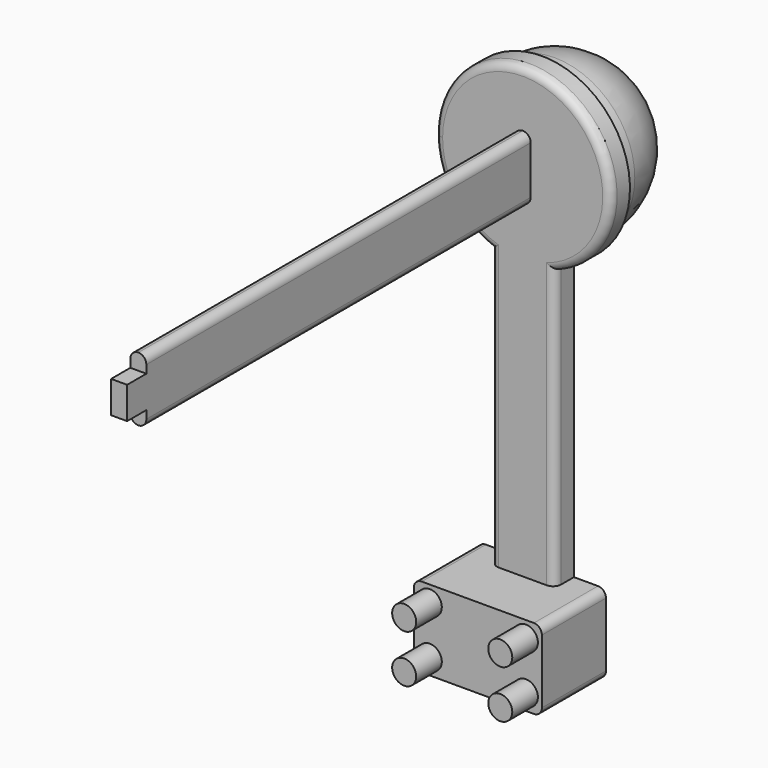
from build123d import *

# Parameters (mm, degrees)
F0_W      = 8
F0_H      = 5
F1_DEPTH  = 5
F2_R      = 0.75
F3_DEPTH  = 2
F4_W      = 4
F4_H      = 1.5
F5_DEPTH  = 23.5
F7_DEPTH  = 1.5
F8_W      = 1
F8_H      = 4
F9_DEPTH  = 30
F10_W     = 1
F10_H     = 2
F11_DEPTH = 1.5
F12_R     = 5
F13_DEPTH = 1
F15_ANGLE = 180
F16_R     = 0.49999
F17_R     = 0.5
F18_R     = 0.5


# Not quite as in the source:
# - a fillet or chamfer is up to 0.001 mm smaller than in the source, because OpenCascade refuses the exact size
# - a feature names something its author has since deleted; it is built from what else it names


with BuildPart() as f1:
    # F0 (on Front) → F1 (new body)
    with BuildSketch(Plane.XZ):
        Rectangle(F0_W, F0_H)
    extrude(amount=F1_DEPTH)

    # F2 (on face) → F3 (join)
    with BuildSketch(Plane.XZ.offset(5)):
        with Locations((-3, 1.5)):
            Circle(F2_R)
        with Locations((3, 1.5)):
            Circle(F2_R)
        with Locations((-3, -1.5)):
            Circle(F2_R)
        with Locations((3, -1.5)):
            Circle(F2_R)
    extrude(amount=F3_DEPTH)

    # F4 (on face) → F5 (join)
    with BuildSketch(Plane.XY.offset(2.5)):
        with Locations((0, -0.75)):
            Rectangle(F4_W, F4_H)
    extrude(amount=F5_DEPTH)

    # F6 (on face) → F7 (join)
    with BuildSketch(Plane(origin=(0, 0, 0), x_dir=(-1, 0, 0), z_dir=(0, 1, 0))):
        with BuildLine():
            ThreePointArc((2, 19.876524617), (4.5414755311, 21.8975815885), (5.5, 25))
            ThreePointArc((5.5, 25), (-3.1024184115, 29.5414755311), (-2, 19.876524617))
            Line((-2, 19.876524617), (-2, 26))
            Line((-2, 26), (2, 26))
            Line((2, 26), (2, 19.876524617))
        make_face()
        with BuildLine():
            Line((-2, 26), (-2, 19.876524617))
            ThreePointArc((-2, 19.876524617), (0, 19.5), (2, 19.876524617))
            Line((2, 19.876524617), (2, 26))
            Line((2, 26), (-2, 26))
        make_face()
    extrude(amount=-F7_DEPTH)

    # F8 (on face) → F9 (join)
    with BuildSketch(Plane.XZ.offset(1.5)):
        with Locations((0, 25)):
            Rectangle(F8_W, F8_H)
    extrude(amount=F9_DEPTH)

    # F10 (on face) → F11 (join)
    with BuildSketch(Plane.XZ.offset(31.5)):
        with Locations((0, 25)):
            Rectangle(F10_W, F10_H)
    extrude(amount=F11_DEPTH)

    # F12 (on face) → F13 (join)
    with BuildSketch(Plane(origin=(0, 0, 0), x_dir=(-1, 0, 0), z_dir=(0, 1, 0))):
        with Locations((0, 25)):
            Circle(F12_R)
    extrude(amount=F13_DEPTH)

    # F14 (on face) → F15 (revolve)
    with BuildSketch(Plane(origin=(0, 1, 0), x_dir=(-1, 0, 0), z_dir=(0, 1, 0))):
        with BuildLine():
            Line((0, 20), (0, 30))
            ThreePointArc((0, 30), (-5, 25), (0, 20))
        make_face()
    revolve(axis=Axis((0, 1, 25), (0, 0, 1)), revolution_arc=F15_ANGLE)

    # F16 (radius 0.5 in the source; OpenCascade refuses exactly that, so slightly less here)
    f16_edges = [f1.edges().sort_by_distance(p)[0] for p in [
        (-0.5, -16.5, 27),
        (0.5, -16.5, 27),
        (0.5, -16.5, 23),
        (-0.5, -16.5, 23),
    ]]
    fillet(f16_edges, radius=F16_R)

    # F17
    f17_edges = [f1.edges().sort_by_distance(p)[0] for p in [
        (-4, -2.5, 2.5),
        (-4, -2.5, -2.5),
        (4, -2.5, -2.5),
        (4, -2.5, 2.5),
    ]]
    fillet(f17_edges, radius=F17_R)

    # F18
    f18_edges = [f1.edges().sort_by_distance(p)[0] for p in [
        (-2, -1.5, 11.188262),
        (2, -1.5, 11.188262),
        (0, -1.5, 30.5),
    ]]
    fillet(f18_edges, radius=F18_R)


solid = f1.part
